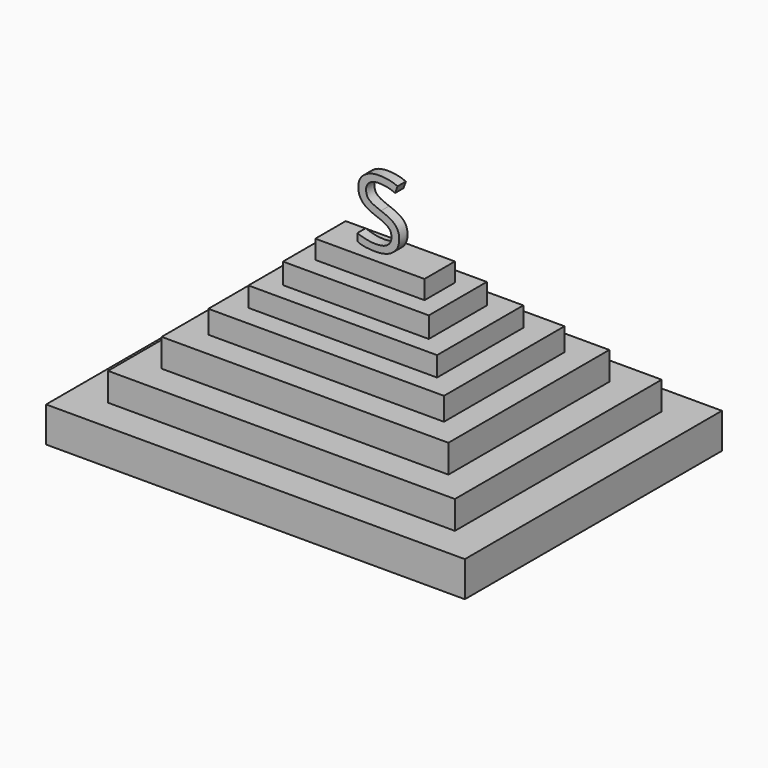
from build123d import *

# Parameters (mm, degrees)
F0_W          = 102.3992821574
F0_H          = 78.5737074912
F1_DEPTH      = 8.636
F2_W          = 84.8258063197
F2_H          = 63.1969161332
F3_DEPTH      = 15.494
F4_W          = 70.1249204576
F4_H          = 49.1719320416
F5_DEPTH      = 22.352
F6_W          = 57.6207172126
F6_H          = 36.8367042392
F7_DEPTH      = 27.94
F8_W          = 46.1303703487
F8_H          = 26.3602118939
F9_DEPTH      = 32.766
F10_W         = 35.6538761407
F10_H         = 17.742450349
F11_DEPTH     = 37.846
F12_W         = 26.6981637105
F12_H         = 9.2936644796
F13_DEPTH     = 42.418
F17_TEXT_SIZE = 22.7647885266
F18_DEPTH     = 2.54


# Not quite as in the source:
# - a feature names something its author has since deleted; it is built from what else it names
# - the program builds the solid bodies; features that only make, move or delete a surface that nothing else refers to are left out
# - Text() gives the source's letters only with a copy of the font that has no kerning and outlines rounded to 1/6400 em; it was checked with that copy


with BuildPart() as f1:
    # F0 (on Top) → F1 (new body)
    with BuildSketch(Plane.XY):
        with Locations((0.3379508853, -1.1828299612)):
            Rectangle(F0_W, F0_H)
    extrude(amount=F1_DEPTH)

    # F2 (on Top) → F3 (join)
    with BuildSketch(Plane.XY):
        with Locations((0.3379508853, -0.9293649346)):
            Rectangle(F2_W, F2_H)
    extrude(amount=F3_DEPTH)

    # F4 (on Top) → F5 (join)
    with BuildSketch(Plane.XY):
        with Locations((0.4224386066, -0.8448790759)):
            Rectangle(F4_W, F4_H)
    extrude(amount=F5_DEPTH)

    # F6 (on Top) → F7 (join)
    with BuildSketch(Plane.XY):
        with Locations((0.5914149806, -0.7603904232)):
            Rectangle(F6_W, F6_H)
    extrude(amount=F7_DEPTH)

    # F8 (on Top) → F9 (join)
    with BuildSketch(Plane.XY):
        with Locations((0.5914140493, -0.9293667972)):
            Rectangle(F8_W, F8_H)
    extrude(amount=F9_DEPTH)

    # F10 (on Top) → F11 (join)
    with BuildSketch(Plane.XY):
        with Locations((0.4224395379, -1.0138540529)):
            Rectangle(F10_W, F10_H)
    extrude(amount=F11_DEPTH)

    # F12 (on Top) → F13 (join)
    with BuildSketch(Plane.XY):
        with Locations((0.337951351, -0.8448784938)):
            Rectangle(F12_W, F12_H)
    extrude(amount=F13_DEPTH)


with BuildPart() as f18:
    # F17 (on Front) → F18 (new body)
    with BuildSketch(Plane.XZ):
        with Locations((-6.2521020882, 42.6663644612)):
            Text('S', F17_TEXT_SIZE, font='Open Sans', text_align=(TextAlign.LEFT, TextAlign.BOTTOM))
    extrude(amount=F18_DEPTH)


solid = Compound([f1.part, f18.part])
